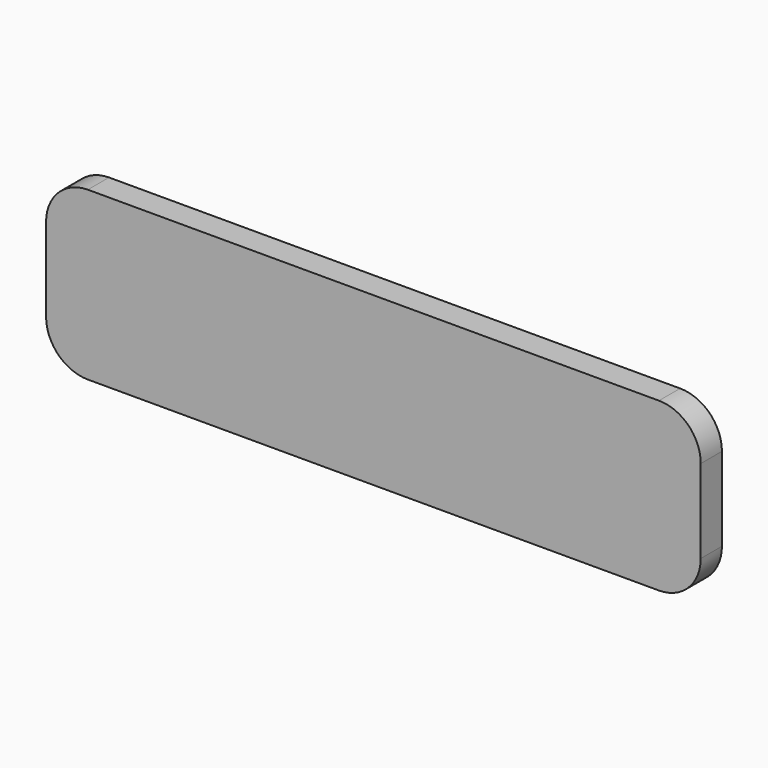
from build123d import *

# Parameters (mm, degrees)
F0_W         = 47
F0_H         = 12
F1_DEPTH     = 1.9
F2_W         = 42.6
F2_H         = 7.6
F3_DEPTH     = 2
F4_T4_DEPTH  = 52.9885099991
F4_T9_DEPTH  = 17.9885099991
F4_T14_DEPTH = 52.9885099991
F4_T19_DEPTH = 17.9885099991
F5_R         = 3


# Not quite as in the source:
# - a fillet or chamfer that OpenCascade refuses, or shapes differently, is made with other operations: its cross-section is extruded or revolved along the edge and cut away or added


with BuildPart() as f1:
    # F0 (on Front) → F1 (new body)
    with BuildSketch(Plane.XZ):
        Rectangle(F0_W, F0_H)
    extrude(amount=F1_DEPTH)

    # F2 (on face) → F3 (join)
    with BuildSketch(Plane(origin=(0, 0, 0), x_dir=(-1, 0, 0), z_dir=(0, 1, 0))):
        Rectangle(F2_W, F2_H)
    extrude(amount=F3_DEPTH)

    # F4: chamfer of 0.5 x 2 on 4 edges, made by hand


with BuildPart() as f4_tool2:
    # F4_s3 → F4_t4 (new body)
    with BuildSketch(Plane.YZ.offset(26.4942549995)):
        Polygon((0, -3.8), (2, -3.3), (2, -3.8), align=None)
    extrude(amount=-F4_T4_DEPTH)

    split(bisect_by=Plane.XZ, keep=Keep.BOTTOM)


with BuildPart() as f1_1:
    add(f1.part)

    # F4_t1: cut F4_tool2
    add(f4_tool2.part, mode=Mode.SUBTRACT)


with BuildPart() as f4_tool7:
    # F4_s8 → F4_t9 (new body)
    with BuildSketch(Plane.XY.offset(-8.9942549995)):
        Polygon((-21.3, 0), (-20.8, 2), (-21.3, 2), align=None)
    extrude(amount=F4_T9_DEPTH)

    split(bisect_by=Plane.XZ, keep=Keep.BOTTOM)


with BuildPart() as f1_2:
    add(f1_1.part)

    # F4_t6: cut F4_tool7
    add(f4_tool7.part, mode=Mode.SUBTRACT)


with BuildPart() as f4_tool12:
    # F4_s13 → F4_t14 (new body)
    with BuildSketch(Plane.YZ.offset(-26.4942549995)):
        Polygon((0, 3.8), (2, 3.3), (2, 3.8), align=None)
    extrude(amount=F4_T14_DEPTH)

    split(bisect_by=Plane.XZ, keep=Keep.BOTTOM)


with BuildPart() as f1_3:
    add(f1_2.part)

    # F4_t11: cut F4_tool12
    add(f4_tool12.part, mode=Mode.SUBTRACT)


with BuildPart() as f4_tool17:
    # F4_s18 → F4_t19 (new body)
    with BuildSketch(Plane.XY.offset(8.9942549995)):
        Polygon((21.3, 0), (20.8, 2), (21.3, 2), align=None)
    extrude(amount=-F4_T19_DEPTH)

    split(bisect_by=Plane.XZ, keep=Keep.BOTTOM)


with BuildPart() as f1_4:
    add(f1_3.part)

    # F4_t16: cut F4_tool17
    add(f4_tool17.part, mode=Mode.SUBTRACT)

    # F5
    f5_edges = [f1_4.edges().sort_by_distance(p)[0] for p in [
        (-23.5, -0.95, -6),
        (23.5, -0.95, -6),
        (23.5, -0.95, 6),
        (-23.5, -0.95, 6),
        (-21.05, 1, 3.55),
        (-21.05, 1, -3.55),
        (21.05, 1, 3.55),
        (21.05, 1, -3.55),
    ]]
    fillet(f5_edges, radius=F5_R)


solid = f1_4.part
